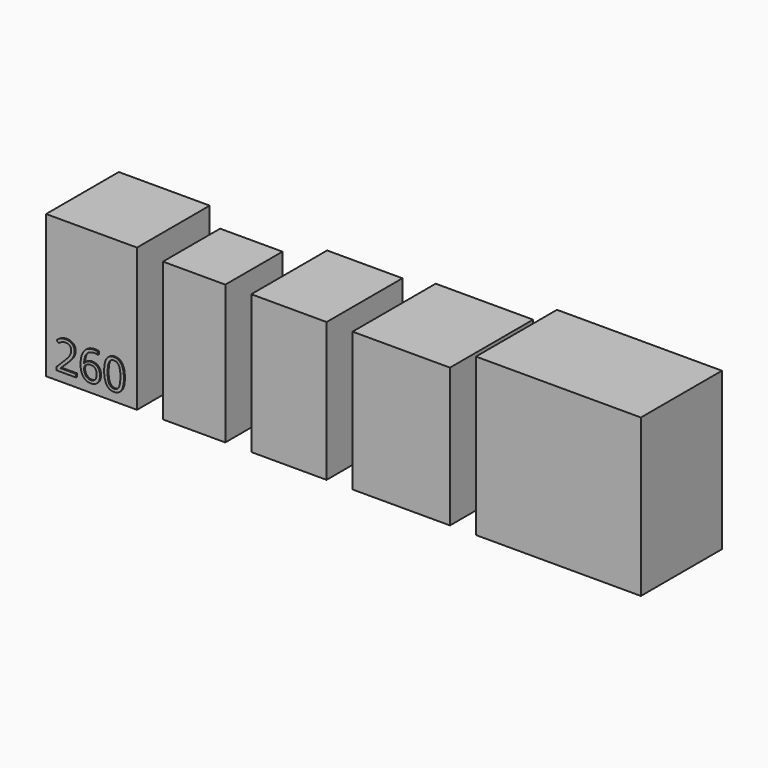
from build123d import *

# Parameters (mm, degrees)
F0_W         = 700
F0_H         = 700
F1_DEPTH     = 1100
F0_W_2       = 480
F0_H_2       = 550
F2_DEPTH     = 1070
F0_W_3       = 580
F0_H_3       = 730
F3_DEPTH     = 1070
F0_W_4       = 750
F0_H_4       = 800
F0_W_5       = 1270
F0_H_5       = 780
F4_DEPTH     = 1210
F5_TEXT_SIZE = 321.7773305045
F6_DEPTH     = 10


# Not quite as in the source:
# - Text() gives the source's letters only with a copy of the font that has no kerning and outlines rounded to 1/6400 em; it was checked with that copy


with BuildPart() as f1:
    # F0 (on Top) → F1 (new body)
    with BuildSketch(Plane.XY):
        with Locations((350, 350)):
            Rectangle(F0_W, F0_H)
    extrude(amount=F1_DEPTH)

    # F5 (on face) → F6 (join)
    with BuildSketch(Plane.XZ):
        with Locations((71.2067857385, 73.3258724213)):
            Text('260', F5_TEXT_SIZE, font='Open Sans', text_align=(TextAlign.LEFT, TextAlign.BOTTOM))
    extrude(amount=F6_DEPTH)


with BuildPart() as f2:
    # F0 (on Top) → F2 (new body)
    with BuildSketch(Plane.XY):
        with Locations((1140, 275)):
            Rectangle(F0_W_2, F0_H_2)
    extrude(amount=F2_DEPTH)


with BuildPart() as f3:
    # F0 (on Top) → F3 (new body)
    with BuildSketch(Plane.XY):
        with Locations((1870, 365)):
            Rectangle(F0_W_3, F0_H_3)
    extrude(amount=F3_DEPTH)


with BuildPart() as f3b:
    # F0 (on Top) → F3, piece 2 (new body)
    with BuildSketch(Plane.XY):
        with Locations((2735, 400)):
            Rectangle(F0_W_4, F0_H_4)
    extrude(amount=F3_DEPTH)


with BuildPart() as f4:
    # F0 (on Top) → F4 (new body)
    with BuildSketch(Plane.XY):
        with Locations((3945, 390)):
            Rectangle(F0_W_5, F0_H_5)
    extrude(amount=F4_DEPTH)


solid = Compound([f1.part, f2.part, f3.part, f3b.part, f4.part])
